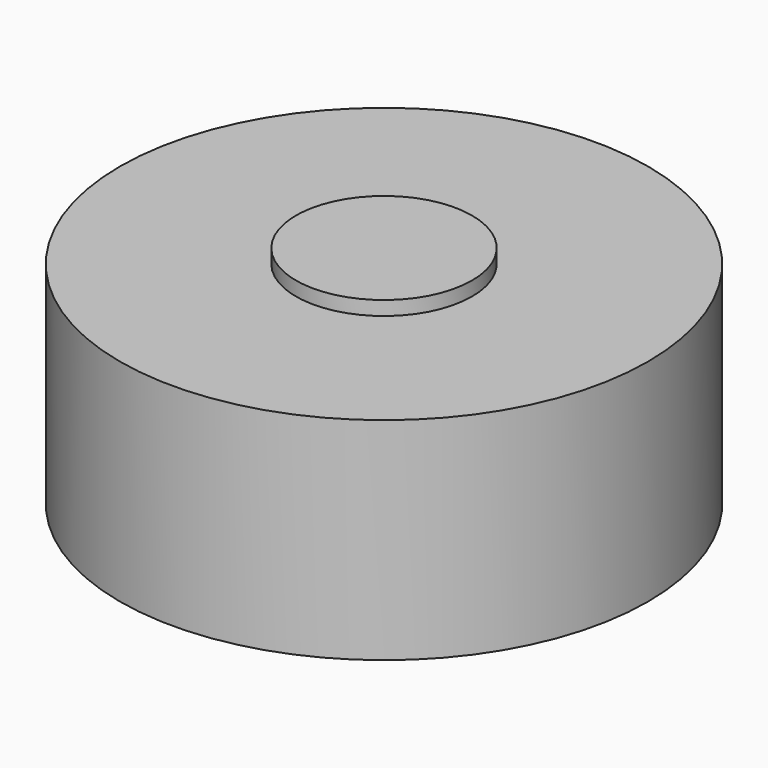
from build123d import *

# Parameters (mm, degrees)
F0_R        = 37.5
F0_R_2      = 30.5
F1_DEPTH    = 40
F2_START    = 20
F0_R_3      = 12.5
F2_DEPTH    = 20
F3_START    = 39
F3_DEPTH    = 3
F4_S5_R     = 30.5
F4_T6_DEPTH = 47
F5_DEPTH    = 10


# Not quite as in the source:
# - a fillet or chamfer that OpenCascade refuses, or shapes differently, is made with other operations: its cross-section is extruded or revolved along the edge and cut away or added


with BuildPart() as f1:
    # F0 (on Top) → F1 (new body)
    with BuildSketch(Plane.XY):
        Circle(F0_R)
        Circle(F0_R_2, mode=Mode.SUBTRACT)
    extrude(amount=F1_DEPTH)

    # F0 (on Top) → F2 (join)
    with BuildSketch(Plane.XY.offset(F2_START)):
        Circle(F0_R_2)
        Circle(F0_R_3, mode=Mode.SUBTRACT)
    extrude(amount=F2_DEPTH)

    # F0 (on Top) → F3 (join)
    with BuildSketch(Plane.XY.offset(F3_START)):
        Circle(F0_R_3)
    extrude(amount=F3_DEPTH)

    # F4: chamfer of 19 on 1 edges, made by hand


with BuildPart() as f4_tool2:
    # F4_s3 → F4_t4 (revolve)
    with BuildSketch(Plane.XZ):
        Polygon((31.5, 20), (12.5, 39), (12.5, 20), align=None)
    revolve(axis=Axis((0, 0, 20), (0, 0, 1)))

    # F4_s5 → F4_t6 (intersect, symmetric)
    with BuildSketch(Plane.XY.offset(29.5)):
        Circle(F4_S5_R)
    extrude(amount=F4_T6_DEPTH, both=True, mode=Mode.INTERSECT)

    split(bisect_by=Plane.XY.offset(39), keep=Keep.BOTTOM)


with BuildPart() as f1_1:
    add(f1.part)

    # F4_t1: cut F4_tool2
    add(f4_tool2.part, mode=Mode.SUBTRACT)

    # F5 (cut): a face of the model
    f5_faces = [f1_1.faces().sort_by_distance(p)[0] for p in [
        (-36.4393398282, 0, 0),
    ]]
    extrude(f5_faces, amount=-F5_DEPTH, mode=Mode.SUBTRACT)


solid = f1_1.part
